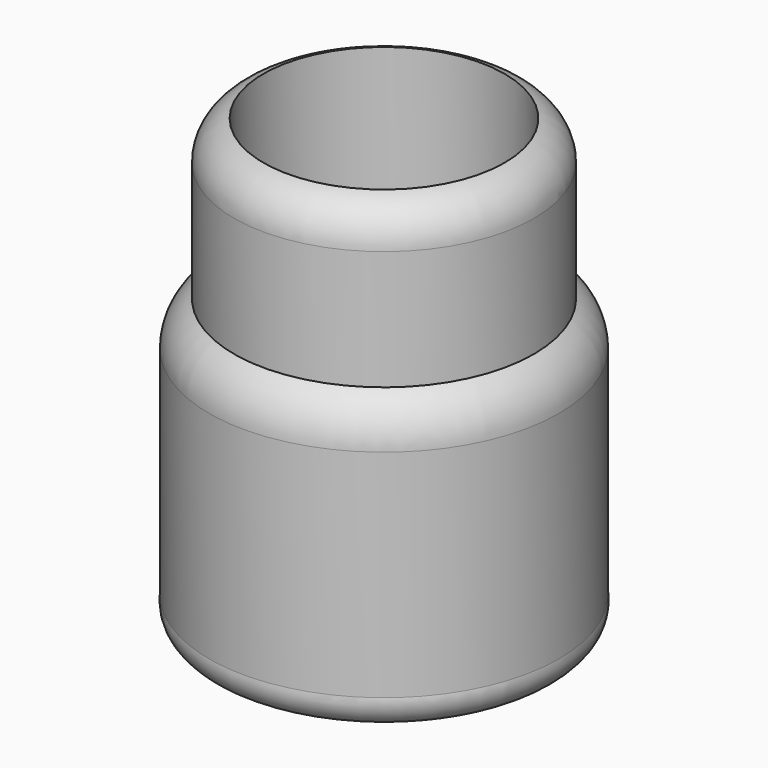
from build123d import *


# Not quite as in the source:
# - a fillet or chamfer that OpenCascade refuses, or shapes differently, is made with other operations: its cross-section is extruded or revolved along the edge and cut away or added


with BuildPart() as f1:
    # F0 (on Front) → F1 (revolve)
    with BuildSketch(Plane.XZ):
        with BuildLine():
            Line((0, 3.4511274384), (0, 0))
            Line((0, 0), (18.3868259192, 0))
            ThreePointArc((18.3868259192, 0), (20.9391502019, 1.1918933999), (21.6636881232, 3.9140274748))
            Line((21.6636881232, 3.9140274748), (21.6636881232, 30.6750517339))
            ThreePointArc((21.6636881232, 30.6750517339), (20.8362073086, 33.8137273466), (18.5688734055, 36.1364856362))
            Line((18.5688734055, 36.1364856362), (18.5688734055, 55.7976476848))
            Line((18.5688734055, 55.7976476848), (14.9279180914, 55.7976476848))
            Line((14.9279180914, 55.7976476848), (14.9279180914, 36.1364856362))
            ThreePointArc((14.9279180914, 36.1364856362), (17.4559954455, 33.877501736), (18.5688734055, 30.6750517339))
            Line((18.5688734055, 30.6750517339), (18.3868259192, 3.3287243314))
            Line((18.3868259192, 3.3287243314), (0, 3.4511274384))
        make_face()
    revolve(axis=Axis((0, 0, 1.7255637192), (0, 0, -1)))

    # F2: fillet of radius 5.08 on 1 edges, made by hand

    # F2_s1 → F2_t2 (revolve, cut)
    with BuildSketch(Plane.XZ):
        with BuildLine():
            ThreePointArc((18.5688734055, 50.9257332365), (17.5580715454, 53.9667900425), (14.9279180914, 55.7976476848))
            Line((14.9279180914, 55.7976476848), (18.5688734055, 55.7976476848))
            Line((18.5688734055, 55.7976476848), (18.5688734055, 50.9257332365))
        make_face()
    revolve(axis=Axis((0, 0, 55.7976476848), (0, 0, -1)), mode=Mode.SUBTRACT)


solid = f1.part
